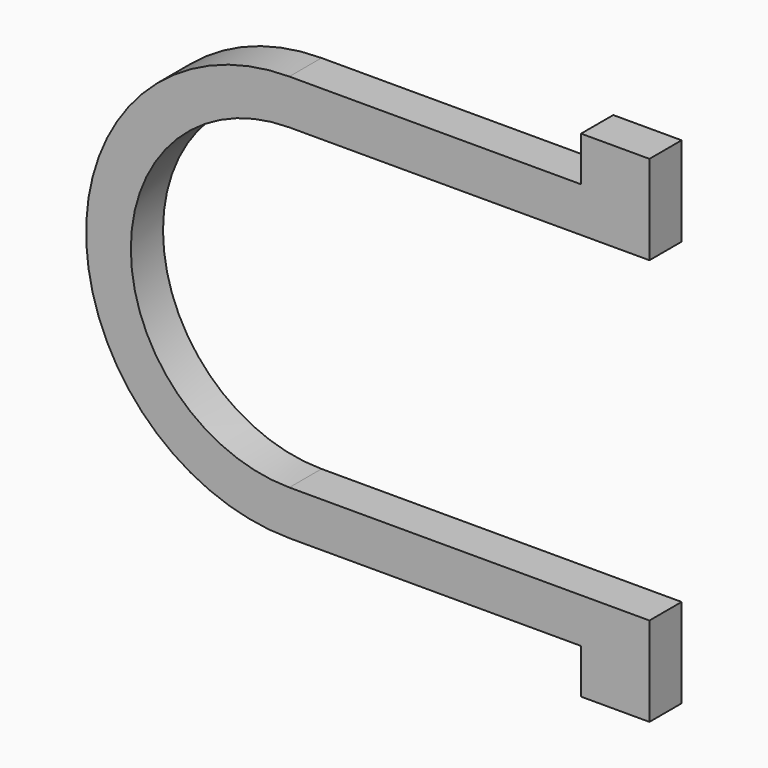
from build123d import *

# Parameters (mm, degrees)
F1_DEPTH = 25.4


# Not quite as in the source:
# - a feature names something its author has since deleted; it is built from what else it names


with BuildPart() as f1:
    # F0 (on Front) → F1 (new body)
    with BuildSketch(Plane.XZ):
        with BuildLine():
            ThreePointArc((3.5129496086, 128.2487611501), (-124.8295958309, -0.0937842894), (3.5129496086, -128.4363297289))
            Line((3.5129496086, -128.4363297289), (187.7788752317, -128.4363297289))
            Line((187.7788752317, -128.4363297289), (187.7788752317, -156.6303297289))
            Line((187.7788752317, -156.6303297289), (230.9588752317, -156.6303297289))
            Line((230.9588752317, -156.6303297289), (230.9588752317, -128.4363297289))
            Line((230.9588752317, -128.4363297289), (230.9588752317, -100.2423297289))
            Line((230.9588752317, -100.2423297289), (3.5129496086, -100.2423297289))
            ThreePointArc((3.5129496086, -100.2423297289), (-96.5909865333, -0.138393587), (3.5129496086, 99.9655425549))
            Line((3.5129496086, 99.9655425549), (230.9588752317, 100.0547611501))
            Line((230.9588752317, 100.0547611501), (230.9588752317, 128.2487611501))
            Line((230.9588752317, 128.2487611501), (230.9588752317, 156.4427611501))
            Line((230.9588752317, 156.4427611501), (187.7788752317, 156.4427611501))
            Line((187.7788752317, 156.4427611501), (187.7788752317, 128.2487611501))
            Line((187.7788752317, 128.2487611501), (3.5129496086, 128.2487611501))
        make_face()
    extrude(amount=F1_DEPTH)


solid = f1.part
